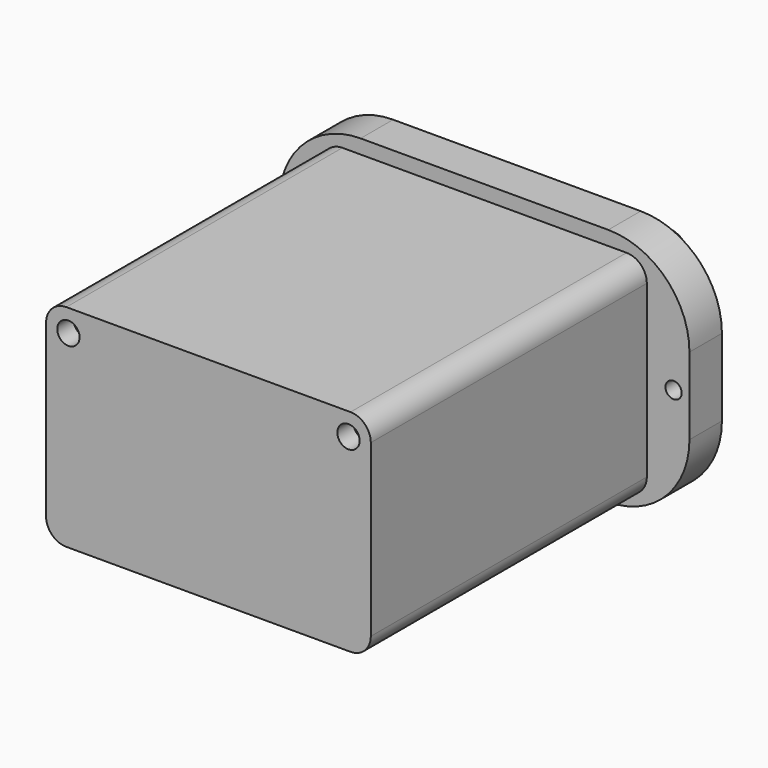
from build123d import *

# Parameters (mm, degrees)
F0_R         = 3.5
F1_DEPTH     = 10
F0_R_2       = 2.75
F2_DEPTH     = 95
F3_DEPTH     = 90
F4_DEPTH     = 3
F5_T1_DEPTH  = 41
F5_T3_DEPTH  = 70
F5_T5_DEPTH  = 42
F5_T7_DEPTH  = 69
F5_T10_ANGLE = 90
F5_T12_ANGLE = 90
F5_T14_ANGLE = 90
F5_T16_ANGLE = 90
F0_R_3       = 2
F6_DEPTH     = 10
F7_DEPTH     = 5


# Not quite as in the source:
# - a fillet or chamfer that OpenCascade refuses, or shapes differently, is made with other operations: its cross-section is extruded or revolved along the edge and cut away or added


with BuildPart() as f1:
    # F0 (on Front) → F1 (new body)
    with BuildSketch(Plane.XZ):
        with BuildLine():
            Line((30.5, 29.5), (-30.5, 29.5))
            ThreePointArc((-30.5, 29.5), (-44.6421356237, 23.6421356237), (-50.5, 9.5))
            Line((-50.5, 9.5), (-50.5, -9.5))
            ThreePointArc((-50.5, -9.5), (-44.6421356237, -23.6421356237), (-30.5, -29.5))
            Line((-30.5, -29.5), (30.5, -29.5))
            ThreePointArc((30.5, -29.5), (44.6421356237, -23.6421356237), (50.5, -9.5))
            Line((50.5, -9.5), (50.5, 9.5))
            ThreePointArc((50.5, 9.5), (44.6421356237, 23.6421356237), (30.5, 29.5))
        make_face()
        with Locations((-46.59, 0)):
            Circle(F0_R, mode=Mode.SUBTRACT)
        with BuildLine():
            ThreePointArc((-40, 21), (-38.5355339059, 24.5355339059), (-35, 26))
            Line((-35, 26), (35, 26))
            ThreePointArc((35, 26), (38.5355339059, 24.5355339059), (40, 21))
            Line((40, 21), (40, -21))
            ThreePointArc((40, -21), (38.5355339059, -24.5355339059), (35, -26))
            Line((35, -26), (-35, -26))
            ThreePointArc((-35, -26), (-38.5355339059, -24.5355339059), (-40, -21))
            Line((-40, -21), (-40, 21))
        make_face(mode=Mode.SUBTRACT)
        with Locations((46.59, 0)):
            Circle(F0_R, mode=Mode.SUBTRACT)
    extrude(amount=F1_DEPTH)

    # F0 (on Front) → F2 (join)
    with BuildSketch(Plane.XZ):
        with BuildLine():
            Line((35, 26), (-35, 26))
            ThreePointArc((-35, 26), (-38.5355339059, 24.5355339059), (-40, 21))
            Line((-40, 21), (-40, -21))
            ThreePointArc((-40, -21), (-38.5355339059, -24.5355339059), (-35, -26))
            Line((-35, -26), (35, -26))
            ThreePointArc((35, -26), (38.5355339059, -24.5355339059), (40, -21))
            Line((40, -21), (40, 21))
            ThreePointArc((40, 21), (38.5355339059, 24.5355339059), (35, 26))
        make_face()
        with BuildLine():
            ThreePointArc((-37.5, 20.5), (-36.6213203436, 22.6213203436), (-34.5, 23.5))
            Line((-34.5, 23.5), (34.5, 23.5))
            ThreePointArc((34.5, 23.5), (36.6213203436, 22.6213203436), (37.5, 20.5))
            Line((37.5, 20.5), (37.5, -21.5))
            ThreePointArc((37.5, -21.5), (36.9142135624, -22.9142135624), (35.5, -23.5))
            Line((35.5, -23.5), (-34.5, -23.5))
            ThreePointArc((-34.5, -23.5), (-36.6213203436, -22.6213203436), (-37.5, -20.5))
            Line((-37.5, -20.5), (-37.5, 20.5))
        make_face(mode=Mode.SUBTRACT)
        with BuildLine():
            Line((34.5, 23.5), (-34.5, 23.5))
            ThreePointArc((-34.5, 23.5), (-36.6213203436, 22.6213203436), (-37.5, 20.5))
            Line((-37.5, 20.5), (-37.5, -20.5))
            ThreePointArc((-37.5, -20.5), (-36.6213203436, -22.6213203436), (-34.5, -23.5))
            Line((-34.5, -23.5), (35.5, -23.5))
            ThreePointArc((35.5, -23.5), (36.9142135624, -22.9142135624), (37.5, -21.5))
            Line((37.5, -21.5), (37.5, 20.5))
            ThreePointArc((37.5, 20.5), (36.6213203436, 22.6213203436), (34.5, 23.5))
        make_face()
        with Locations((-34.5, 20.5)):
            Circle(F0_R_2, mode=Mode.SUBTRACT)
        with Locations((34.5, 20.5)):
            Circle(F0_R_2, mode=Mode.SUBTRACT)
    extrude(amount=F2_DEPTH)

    # F0 (on Front) → F3 (cut)
    with BuildSketch(Plane.XZ):
        with BuildLine():
            Line((34.5, 23.5), (-34.5, 23.5))
            ThreePointArc((-34.5, 23.5), (-36.6213203436, 22.6213203436), (-37.5, 20.5))
            Line((-37.5, 20.5), (-37.5, -20.5))
            ThreePointArc((-37.5, -20.5), (-36.6213203436, -22.6213203436), (-34.5, -23.5))
            Line((-34.5, -23.5), (35.5, -23.5))
            ThreePointArc((35.5, -23.5), (36.9142135624, -22.9142135624), (37.5, -21.5))
            Line((37.5, -21.5), (37.5, 20.5))
            ThreePointArc((37.5, 20.5), (36.6213203436, 22.6213203436), (34.5, 23.5))
        make_face()
        with Locations((-34.5, 20.5)):
            Circle(F0_R_2, mode=Mode.SUBTRACT)
        with Locations((34.5, 20.5)):
            Circle(F0_R_2, mode=Mode.SUBTRACT)
    extrude(amount=F3_DEPTH, mode=Mode.SUBTRACT)

    # F0 (on Front) → F4 (join)
    with BuildSketch(Plane.XZ):
        with BuildLine():
            Line((35, 26), (-35, 26))
            ThreePointArc((-35, 26), (-38.5355339059, 24.5355339059), (-40, 21))
            Line((-40, 21), (-40, -21))
            ThreePointArc((-40, -21), (-38.5355339059, -24.5355339059), (-35, -26))
            Line((-35, -26), (35, -26))
            ThreePointArc((35, -26), (38.5355339059, -24.5355339059), (40, -21))
            Line((40, -21), (40, 21))
            ThreePointArc((40, 21), (38.5355339059, 24.5355339059), (35, 26))
        make_face()
        with BuildLine():
            ThreePointArc((-37.5, 20.5), (-36.6213203436, 22.6213203436), (-34.5, 23.5))
            Line((-34.5, 23.5), (34.5, 23.5))
            ThreePointArc((34.5, 23.5), (36.6213203436, 22.6213203436), (37.5, 20.5))
            Line((37.5, 20.5), (37.5, -21.5))
            ThreePointArc((37.5, -21.5), (36.9142135624, -22.9142135624), (35.5, -23.5))
            Line((35.5, -23.5), (-34.5, -23.5))
            ThreePointArc((-34.5, -23.5), (-36.6213203436, -22.6213203436), (-37.5, -20.5))
            Line((-37.5, -20.5), (-37.5, 20.5))
        make_face(mode=Mode.SUBTRACT)
    extrude(amount=-F4_DEPTH)

    # F5: fillet of radius 3 on 2 edges, made by hand

    # F5_s2 → F5_t1 (cut)
    with BuildSketch(Plane.XY.offset(-20.5)):
        with BuildLine():
            ThreePointArc((-40.5, 3), (-38.3786796564, 2.1213203436), (-37.5, 0))
            Line((-37.5, 0), (-37.5, 3))
            Line((-37.5, 3), (-40.5, 3))
        make_face()
    extrude(amount=F5_T1_DEPTH, mode=Mode.SUBTRACT)

    # F5_s4 → F5_t3 (cut)
    with BuildSketch(Plane.YZ.offset(-34.5)):
        with BuildLine():
            ThreePointArc((3, -26.5), (2.1213203436, -24.3786796564), (0, -23.5))
            Line((0, -23.5), (3, -23.5))
            Line((3, -23.5), (3, -26.5))
        make_face()
    extrude(amount=F5_T3_DEPTH, mode=Mode.SUBTRACT)

    # F5_s6 → F5_t5 (cut)
    with BuildSketch(Plane.XY.offset(-21.5)):
        with BuildLine():
            ThreePointArc((40.5, 3), (38.3786796564, 2.1213203436), (37.5, 0))
            Line((37.5, 0), (37.5, 3))
            Line((37.5, 3), (40.5, 3))
        make_face()
    extrude(amount=F5_T5_DEPTH, mode=Mode.SUBTRACT)

    # F5_s8 → F5_t7 (cut)
    with BuildSketch(Plane.YZ.offset(-34.5)):
        with BuildLine():
            ThreePointArc((3, 26.5), (2.1213203436, 24.3786796564), (0, 23.5))
            Line((0, 23.5), (3, 23.5))
            Line((3, 23.5), (3, 26.5))
        make_face()
    extrude(amount=F5_T7_DEPTH, mode=Mode.SUBTRACT)

    # F5_s9 → F5_t10 (revolve, cut)
    with BuildSketch(Plane.XY.offset(-21.5)):
        with BuildLine():
            ThreePointArc((40.5, 3), (38.3786796564, 2.1213203436), (37.5, 0))
            Line((37.5, 0), (37.5, 3))
            Line((37.5, 3), (40.5, 3))
        make_face()
    revolve(axis=Axis((35.5, 3, -21.5), (0, 1, 0)), revolution_arc=F5_T10_ANGLE, mode=Mode.SUBTRACT)

    # F5_s11 → F5_t12 (revolve, cut)
    with BuildSketch(Plane.YZ.offset(-34.5)):
        with BuildLine():
            ThreePointArc((3, -26.5), (2.1213203436, -24.3786796564), (0, -23.5))
            Line((0, -23.5), (3, -23.5))
            Line((3, -23.5), (3, -26.5))
        make_face()
    revolve(axis=Axis((-34.5, 3, -20.5), (0, 1, 0)), revolution_arc=F5_T12_ANGLE, mode=Mode.SUBTRACT)

    # F5_s13 → F5_t14 (revolve, cut)
    with BuildSketch(Plane.YZ.offset(34.5)):
        with BuildLine():
            ThreePointArc((0, 23.5), (2.1213203436, 24.3786796564), (3, 26.5))
            Line((3, 26.5), (3, 23.5))
            Line((3, 23.5), (0, 23.5))
        make_face()
    revolve(axis=Axis((34.5, 3, 20.5), (0, 1, 0)), revolution_arc=F5_T14_ANGLE, mode=Mode.SUBTRACT)

    # F5_s15 → F5_t16 (revolve, cut)
    with BuildSketch(Plane.XY.offset(20.5)):
        with BuildLine():
            ThreePointArc((-40.5, 3), (-38.3786796564, 2.1213203436), (-37.5, 0))
            Line((-37.5, 0), (-37.5, 3))
            Line((-37.5, 3), (-40.5, 3))
        make_face()
    revolve(axis=Axis((-34.5, 3, 20.5), (0, 1, 0)), revolution_arc=F5_T16_ANGLE, mode=Mode.SUBTRACT)

    # F0 (on Front) → F6 (join)
    with BuildSketch(Plane.XZ):
        with Locations((46.59, 0)):
            Circle(F0_R)
        with Locations((46.59, 0)):
            Circle(F0_R_3, mode=Mode.SUBTRACT)
        with Locations((-46.59, 0)):
            Circle(F0_R)
        with Locations((-46.59, 0)):
            Circle(F0_R_3, mode=Mode.SUBTRACT)
    extrude(amount=F6_DEPTH)

    # F0 (on Front) → F7 (cut)
    with BuildSketch(Plane.XZ):
        with Locations((46.59, 0)):
            Circle(F0_R)
        with Locations((46.59, 0)):
            Circle(F0_R_3, mode=Mode.SUBTRACT)
        with Locations((-46.59, 0)):
            Circle(F0_R)
        with Locations((-46.59, 0)):
            Circle(F0_R_3, mode=Mode.SUBTRACT)
    extrude(amount=F7_DEPTH, mode=Mode.SUBTRACT)


solid = f1.part
